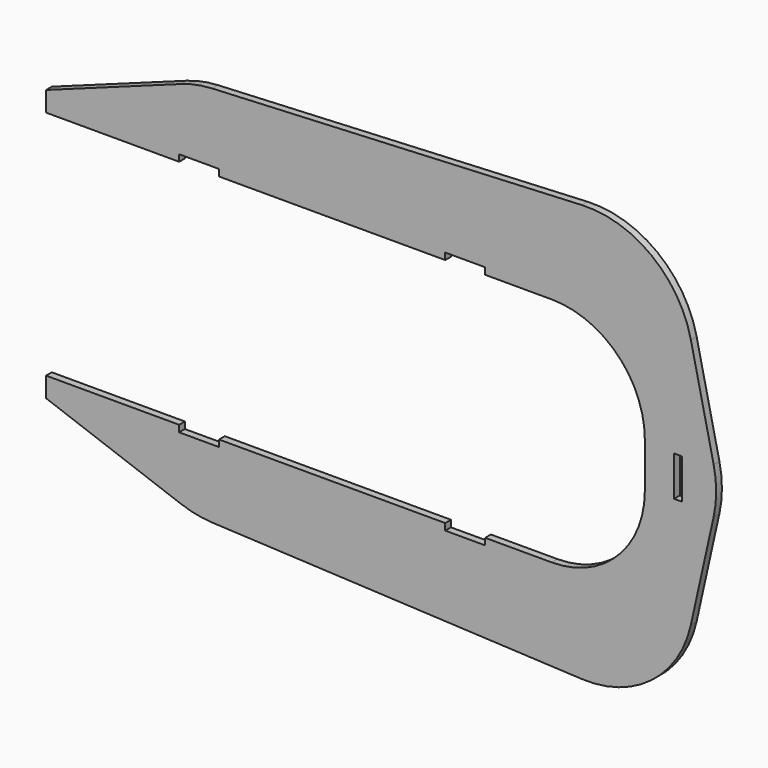
from build123d import *

# Parameters (mm, degrees)
F0_W     = 3.81
F0_H     = 19.05
F1_DEPTH = 3.429


# Not quite as in the source:
# - ends of sketch curves that miss each other by under 0.0002 mm in the source are joined


with BuildPart() as f1:
    # F0 (on Front) → F1 (new body)
    with BuildSketch(Plane.XZ):
        with BuildLine():
            Line((641.7700144, 153.9733014), (749.7200144, 153.9733014))
            Line((749.7200144, 153.9733014), (749.7200144, 157.1483014))
            Line((749.7200144, 157.1483014), (768.7700144, 157.1483014))
            Line((768.7700144, 157.1483014), (768.7700144, 153.9733014))
            Line((768.7700144, 153.9733014), (800.5200144, 153.9733014))
            ThreePointArc((800.5200144, 153.9733014), (831.9509108237, 140.9541978237), (844.9700144, 109.5233014))
            Line((844.9700144, 109.5233014), (844.9700144, 87.9333014))
            ThreePointArc((844.9700144, 87.9333014), (831.9509108237, 56.5024049763), (800.5200144, 43.4833014))
            Line((800.5200144, 43.4833014), (768.7700144, 43.4833014))
            Line((768.7700144, 43.4833014), (768.7700144, 40.3083014))
            Line((768.7700144, 40.3083014), (749.7200144, 40.3083014))
            Line((749.7200144, 40.3083014), (749.7200144, 43.4833014))
            Line((749.7200144, 43.4833014), (641.7700144, 43.4833014))
            Line((641.7700144, 43.4833014), (641.7700144, 40.3083014))
            Line((641.7700144, 40.3083014), (622.7200144, 40.3083014))
            Line((622.7200144, 40.3083014), (622.7200144, 43.4833014))
            Line((622.7200144, 43.4833014), (559.2200144, 43.4833014))
            Line((559.2200144, 43.4833014), (559.2200144, 33.9583014))
            Line((559.2200144, 33.9583014), (623.5700762, 10.5367836))
            ThreePointArc((623.5700762, 10.5367836), (630.9394695232, 8.4681877562), (638.536009535, 7.5302985912))
            Line((638.536009535, 7.5302985912), (814.9544788, -0.844042))
            ThreePointArc((814.9544788, -0.844042), (848.1989075574, 9.5280670864), (866.95206277, 38.8724395401))
            Line((866.95206277, 38.8724395401), (877.8095982, 87.7019074))
            ThreePointArc((877.8095982, 87.7019074), (879.0206956, 98.7282890028), (877.80959757, 109.7546698599))
            Line((877.80959757, 109.7546698599), (866.9520634, 158.5841634))
            ThreePointArc((866.9520634, 158.5841634), (848.1988981839, 187.9285174732), (814.954479338, 198.3006334659))
            Line((814.954479338, 198.3006334659), (638.5360102, 189.9262902))
            ThreePointArc((638.5360102, 189.9262902), (630.9394701135, 188.9883897624), (623.5700733762, 186.9198015582))
            Line((623.5700733762, 186.9198015582), (559.2200144, 163.4983014))
            Line((559.2200144, 163.4983014), (559.2200144, 153.9733014))
            Line((559.2200144, 153.9733014), (622.7200144, 153.9733014))
            Line((622.7200144, 153.9733014), (622.7200144, 157.1483014))
            Line((622.7200144, 157.1483014), (641.7700144, 157.1483014))
            Line((641.7700144, 157.1483014), (641.7700144, 153.9733014))
        make_face()
        with Locations((860.8450144, 98.7283014)):
            Rectangle(F0_W, F0_H, mode=Mode.SUBTRACT)
    extrude(amount=F1_DEPTH)


solid = f1.part
